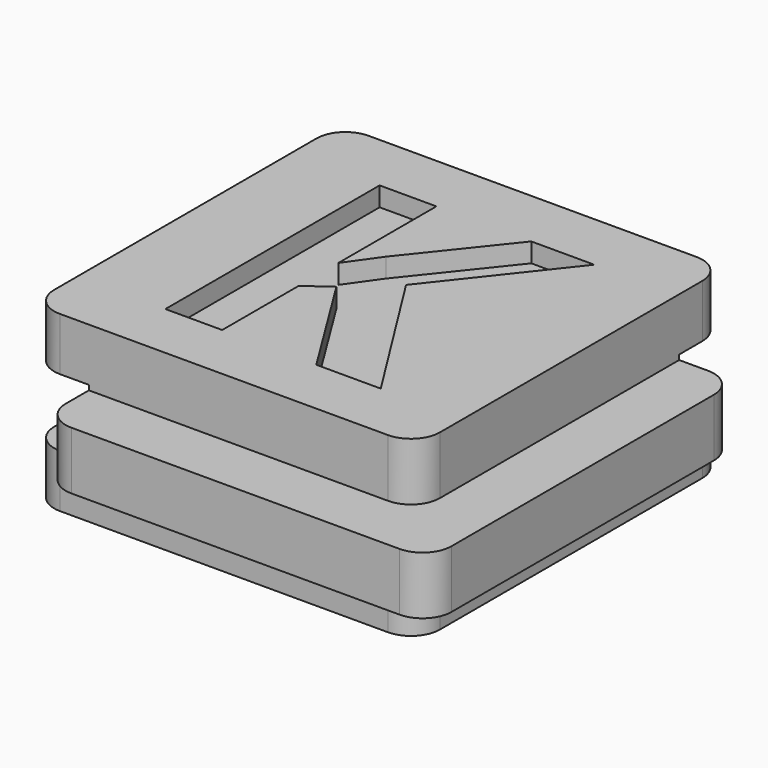
from build123d import *

# Parameters (mm, degrees)
F0_W         = 14
F0_H         = 3
F0_W_2       = 3
F1_DEPTH     = 20
F2_DEPTH     = 3
F3_W         = 3
F3_H         = 3
F4_DEPTH     = 100
F5_W         = 3
F5_H         = 3.5
F6_DEPTH     = 100
F7_R         = 1.5
F8_TEXT_SIZE = 19.4444444444
F9_DEPTH     = 1


# Not quite as in the source:
# - Text() gives the source's letters only with a copy of the font that has no kerning and outlines rounded to 1/6400 em; it was checked with that copy


with BuildPart() as f1:
    # F0 (on Front) → F1 (new body)
    with BuildSketch(Plane.XZ):
        Polygon((10, 1.5), (10, 4.5), (-10, 4.5), (-10, 1.5), (-7, 1.5), (7, 1.5), align=None)
        Rectangle(F0_W, F0_H)
        with Locations((11.5, 0)):
            Rectangle(F0_W_2, F0_H)
        with Locations((8.5, 0)):
            Rectangle(F0_W_2, F0_H)
        with Locations((-8.5, 0)):
            Rectangle(F0_W_2, F0_H)
        Polygon((10, -4.5), (10, -1.5), (7, -1.5), (-7, -1.5), (-10, -1.5), (-10, -4.5), align=None)
    extrude(amount=-F1_DEPTH)

    # F0 (on Front) → F2 (join)
    with BuildSketch(Plane.XZ):
        with Locations((-8.5, 0)):
            Rectangle(F0_W_2, F0_H)
        Rectangle(F0_W, F0_H)
        with Locations((8.5, 0)):
            Rectangle(F0_W_2, F0_H)
        with Locations((11.5, 0)):
            Rectangle(F0_W_2, F0_H)
    extrude(amount=F2_DEPTH)

    # F3 (on face) → F4 (cut)
    with BuildSketch(Plane.YZ.offset(13)):
        Polygon((23, -1.75), (23, 1.75), (17, 1.75), (17, 1.5), (20, 1.5), (20, -1.5), (17, -1.5), (17, -1.75), align=None)
        with Locations((18.5, 0)):
            Rectangle(F3_W, F3_H)
    extrude(amount=-F4_DEPTH, mode=Mode.SUBTRACT)

    # F5 (on face) → F6 (cut)
    with BuildSketch(Plane(origin=(0, 17, 0), x_dir=(-1, 0, 0), z_dir=(0, 1, 0))):
        with Locations((11.5, 0)):
            Rectangle(F5_W, F5_H)
        with Locations((8.5, 0)):
            Rectangle(F5_W, F5_H)
    extrude(amount=-F6_DEPTH, mode=Mode.SUBTRACT)

    # F7
    f7_edges = [f1.edges().sort_by_distance(p)[0] for p in [
        (-7, -3, 0),
        (13, -3, 0),
        (10, 0, 3),
        (10, 0, -3),
        (-10, 0, -3.125),
        (-10, 0, 3.125),
        (-7, 17, 0),
        (-10, 20, 3.125),
        (-10, 20, -3.125),
        (13, 17, 0),
        (10, 20, 3.125),
        (10, 20, -3.125),
    ]]
    fillet(f7_edges, radius=F7_R)

    # F8 (on face) → F9 (cut)
    with BuildSketch(Plane.XY.offset(4.5)):
        with Locations((-7.1801951318, 3)):
            Text('K', F8_TEXT_SIZE, font='Open Sans', font_style=FontStyle.BOLD, text_align=(TextAlign.LEFT, TextAlign.BOTTOM))
    extrude(amount=-F9_DEPTH, mode=Mode.SUBTRACT)


solid = f1.part
